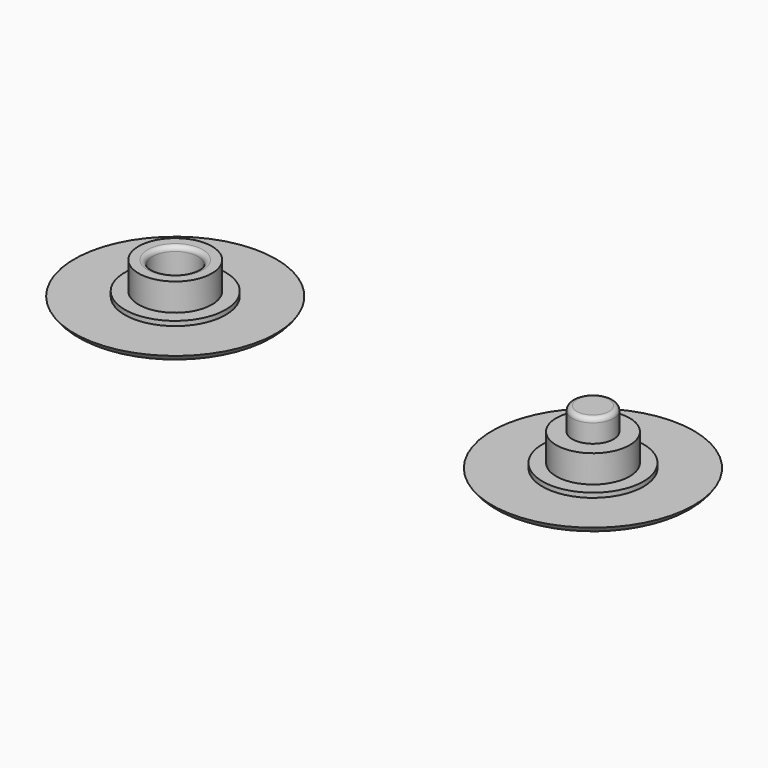
from build123d import *

# Parameters (mm, degrees)
F0_R      = 11
F1_DEPTH  = 1
F2_R      = 5.5
F3_DEPTH  = 0.5
F4_R      = 4
F5_DEPTH  = 3
F7_R      = 2.5
F8_DEPTH  = 3
F9_R      = 5.5
F10_DEPTH = 0.5
F11_R     = 4
F12_DEPTH = 3
F13_R     = 2.25
F14_DEPTH = 2.5
F15_R     = 0.5
F15_2_R   = 0.5


# Not quite as in the source:
# - a fillet or chamfer that OpenCascade refuses, or shapes differently, is made with other operations: its cross-section is extruded or revolved along the edge and cut away or added


with BuildPart() as f1:
    # F0 (on Top) → F1 (new body)
    with BuildSketch(Plane.XY):
        with Locations((-53.6903738976, 42.7074432373)):
            Circle(F0_R)
    extrude(amount=F1_DEPTH)

    # F2 (on face) → F3 (join)
    with BuildSketch(Plane.XY.offset(1)):
        with Locations((-53.6903738976, 42.7074432373)):
            Circle(F2_R)
    extrude(amount=F3_DEPTH)

    # F4 (on face) → F5 (join)
    with BuildSketch(Plane.XY.offset(1.5)):
        with Locations((-53.6903738976, 42.7074432373)):
            Circle(F4_R)
    extrude(amount=F5_DEPTH)

    # F6: fillet of radius 2 on 1 edges, made by hand

    # F6_s1 → F6_t2 (revolve, cut)
    with BuildSketch(Plane.XZ.offset(-42.7074432373)):
        with BuildLine():
            ThreePointArc((-42.6903738976, 1), (-43.4224247051, 0.2679491924), (-44.4224247051, 0))
            Line((-44.4224247051, 0), (-42.6903738976, 0))
            Line((-42.6903738976, 0), (-42.6903738976, 1))
        make_face()
    revolve(axis=Axis((-53.6903738976, 42.7074432373, 0), (0, 0, 1)), mode=Mode.SUBTRACT)

    # F7 (on face) → F8 (cut)
    with BuildSketch(Plane.XY.offset(4.5)):
        with Locations((-53.6903738976, 42.7074432373)):
            Circle(F7_R)
    extrude(amount=-F8_DEPTH, mode=Mode.SUBTRACT)

    # F15
    f15_edges = [f1.edges().sort_by_distance(p)[0] for p in [
        (-56.190374, 42.707443, 4.5),
    ]]
    fillet(f15_edges, radius=F15_R)


with BuildPart() as f1b:
    # F0 (on Top) → F1, piece 2 (new body)
    with BuildSketch(Plane.XY):
        with Locations((-6.1243791133, 40.1936098933)):
            Circle(F0_R)
    extrude(amount=F1_DEPTH)

    # F9 (on face) → F10 (join)
    with BuildSketch(Plane.XY.offset(1)):
        with Locations((-6.1243791133, 40.1936098933)):
            Circle(F9_R)
    extrude(amount=F10_DEPTH)

    # F11 (on face) → F12 (join)
    with BuildSketch(Plane.XY.offset(1.5)):
        with Locations((-6.1243791133, 40.1936098933)):
            Circle(F11_R)
    extrude(amount=F12_DEPTH)

    # F13 (on face) → F14 (join)
    with BuildSketch(Plane.XY.offset(4.5)):
        with Locations((-6.1243791133, 40.1936098933)):
            Circle(F13_R)
    extrude(amount=F14_DEPTH)

    # F15#2
    f15_2_edges = [f1b.edges().sort_by_distance(p)[0] for p in [
        (-8.374379, 40.19361, 7),
    ]]
    fillet(f15_2_edges, radius=F15_2_R)

    # F16: fillet of radius 2 on 1 edges, made by hand

    # F16_s1 → F16_t2 (revolve, cut)
    with BuildSketch(Plane.XZ.offset(-40.1936098933)):
        with BuildLine():
            ThreePointArc((4.8756208867, 1), (4.1435700791, 0.2679491924), (3.1435700791, 0))
            Line((3.1435700791, 0), (4.8756208867, 0))
            Line((4.8756208867, 0), (4.8756208867, 1))
        make_face()
    revolve(axis=Axis((-6.1243791133, 40.1936098933, 0), (0, 0, 1)), mode=Mode.SUBTRACT)


solid = Compound([f1.part, f1b.part])
